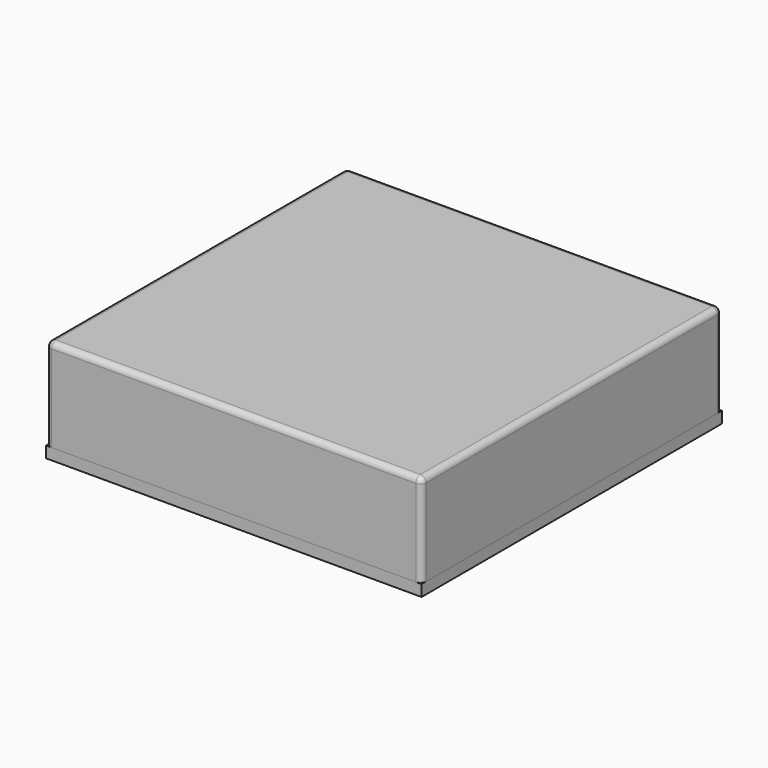
from build123d import *

# Parameters (mm, degrees)
F0_W     = 39.8
F0_H     = 39.8
F0_W_2   = 37.4
F0_H_2   = 37.4
F0_W_3   = 16.9
F0_H_3   = 16.9
F1_DEPTH = 1.2
F2_DEPTH = 10
F3_START = 1.2
F3_DEPTH = 9.8
F4_START = 10
F4_DEPTH = 1
F5_R     = 0.6


with BuildPart() as f1:
    # F0 (on Top) → F1 (new body)
    with BuildSketch(Plane.XY):
        with Locations((-19.9, 37.0918591321)):
            Rectangle(F0_W, F0_H)
        with Locations((-19.9, 37.0918591321)):
            Rectangle(F0_W_2, F0_H_2, mode=Mode.SUBTRACT)
        with Locations((-19.9, 37.0918591321)):
            Rectangle(F0_W_2, F0_H_2)
        Polygon((-37.4, 37.6918591321), (-37.4, 54.5918591321), (-20.5, 54.5918591321), (-19.3, 54.5918591321), (-2.4, 54.5918591321), (-2.4, 37.6918591321), (-2.4, 36.4918591321), (-2.4, 19.5918591321), (-19.3, 19.5918591321), (-20.5, 19.5918591321), (-37.4, 19.5918591321), (-37.4, 36.4918591321), align=None, mode=Mode.SUBTRACT)
        with Locations((-10.85, 46.1418591321)):
            Rectangle(F0_W_3, F0_H_3)
        with Locations((-28.95, 28.0418591321)):
            Rectangle(F0_W_3, F0_H_3)
        with Locations((-28.95, 46.1418591321)):
            Rectangle(F0_W_3, F0_H_3)
        with Locations((-10.85, 28.0418591321)):
            Rectangle(F0_W_3, F0_H_3)
        Polygon((-19.3, 54.5918591321), (-20.5, 54.5918591321), (-20.5, 37.6918591321), (-37.4, 37.6918591321), (-37.4, 36.4918591321), (-20.5, 36.4918591321), (-20.5, 19.5918591321), (-19.3, 19.5918591321), (-19.3, 36.4918591321), (-2.4, 36.4918591321), (-2.4, 37.6918591321), (-19.3, 37.6918591321), align=None)
    extrude(amount=F1_DEPTH)

    # F0 (on Top) → F2 (join)
    with BuildSketch(Plane.XY):
        with Locations((-19.9, 37.0918591321)):
            Rectangle(F0_W_2, F0_H_2)
        Polygon((-37.4, 37.6918591321), (-37.4, 54.5918591321), (-20.5, 54.5918591321), (-19.3, 54.5918591321), (-2.4, 54.5918591321), (-2.4, 37.6918591321), (-2.4, 36.4918591321), (-2.4, 19.5918591321), (-19.3, 19.5918591321), (-20.5, 19.5918591321), (-37.4, 19.5918591321), (-37.4, 36.4918591321), align=None, mode=Mode.SUBTRACT)
        Polygon((-19.3, 54.5918591321), (-20.5, 54.5918591321), (-20.5, 37.6918591321), (-37.4, 37.6918591321), (-37.4, 36.4918591321), (-20.5, 36.4918591321), (-20.5, 19.5918591321), (-19.3, 19.5918591321), (-19.3, 36.4918591321), (-2.4, 36.4918591321), (-2.4, 37.6918591321), (-19.3, 37.6918591321), align=None)
    extrude(amount=F2_DEPTH)


with BuildPart() as f3:
    # F0 (on Top) → F3 (new body)
    with BuildSketch(Plane.XY.offset(F3_START)):
        with Locations((-19.9, 37.0918591321)):
            Rectangle(F0_W, F0_H)
        with Locations((-19.9, 37.0918591321)):
            Rectangle(F0_W_2, F0_H_2, mode=Mode.SUBTRACT)
    extrude(amount=F3_DEPTH)

    # F0 (on Top) → F4 (join)
    with BuildSketch(Plane.XY.offset(F4_START)):
        with Locations((-19.9, 37.0918591321)):
            Rectangle(F0_W, F0_H)
        with Locations((-19.9, 37.0918591321)):
            Rectangle(F0_W_2, F0_H_2, mode=Mode.SUBTRACT)
        with Locations((-19.9, 37.0918591321)):
            Rectangle(F0_W_2, F0_H_2)
        Polygon((-37.4, 37.6918591321), (-37.4, 54.5918591321), (-20.5, 54.5918591321), (-19.3, 54.5918591321), (-2.4, 54.5918591321), (-2.4, 37.6918591321), (-2.4, 36.4918591321), (-2.4, 19.5918591321), (-19.3, 19.5918591321), (-20.5, 19.5918591321), (-37.4, 19.5918591321), (-37.4, 36.4918591321), align=None, mode=Mode.SUBTRACT)
        with Locations((-28.95, 46.1418591321)):
            Rectangle(F0_W_3, F0_H_3)
        with Locations((-10.85, 46.1418591321)):
            Rectangle(F0_W_3, F0_H_3)
        with Locations((-10.85, 28.0418591321)):
            Rectangle(F0_W_3, F0_H_3)
        with Locations((-28.95, 28.0418591321)):
            Rectangle(F0_W_3, F0_H_3)
        Polygon((-19.3, 54.5918591321), (-20.5, 54.5918591321), (-20.5, 37.6918591321), (-37.4, 37.6918591321), (-37.4, 36.4918591321), (-20.5, 36.4918591321), (-20.5, 19.5918591321), (-19.3, 19.5918591321), (-19.3, 36.4918591321), (-2.4, 36.4918591321), (-2.4, 37.6918591321), (-19.3, 37.6918591321), align=None)
    extrude(amount=F4_DEPTH)

    # F5
    f5_edges = [f3.edges().sort_by_distance(p)[0] for p in [
        (-19.9, 56.991859, 11),
        (-39.8, 37.091859, 11),
        (-19.9, 17.191859, 11),
        (0, 37.091859, 11),
        (-39.8, 56.991859, 6.1),
        (-39.8, 17.191859, 6.1),
        (0, 17.191859, 6.1),
        (0, 56.991859, 6.1),
    ]]
    fillet(f5_edges, radius=F5_R)


solid = Compound([f1.part, f3.part])
